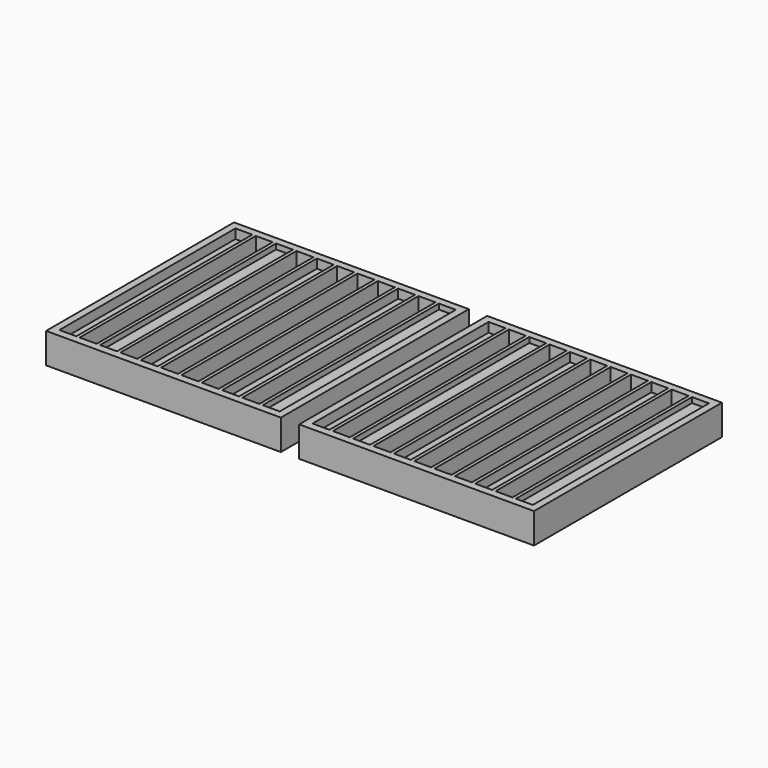
from build123d import *

# Parameters (mm, degrees)
F0_W     = 44.6
F0_H     = 55.1762282848
F0_H_2   = 34.8895229399
F0_H_3   = 66.0242550075
F0_H_4   = 3.5007570405
F0_H_5   = 56.2235750258
F0_H_6   = 10.0867319852
F1_DEPTH = 580
F0_H_7   = 24.8237717152
F0_H_8   = 45.1104770601
F0_H_9   = 13.9757449925
F0_H_10  = 76.4992429595
F0_H_11  = 23.7764249742
F0_H_12  = 69.9132680148
F2_DEPTH = 9
F3_START = 580
F3_DEPTH = 10
F4_W     = 618.6
F4_H     = 619
F4_W_2   = 598.6
F4_H_2   = 599
F5_DEPTH = 80


# Not quite as in the source:
# - a feature names something its author has since deleted; it is built from what else it names


with BuildPart() as f1:
    # F0 (on Front) → F1 (new body)
    with BuildSketch(Plane.XZ):
        Polygon((0, 80), (0, 0), (9, 0), (9, 55.1762282848), (9, 80), align=None)
        with Locations((31.3, 27.5881141424)):
            Rectangle(F0_W, F0_H)
        Polygon((53.6, 55.1762282848), (53.6, 0), (62.6, 0), (62.6, 34.8895229399), (62.6, 80), (53.6, 80), align=None)
        with Locations((84.9, 17.44476147)):
            Rectangle(F0_W, F0_H_2)
        Polygon((107.2, 34.8895229399), (107.2, 0), (116.2, 0), (116.2, 66.0242550075), (116.2, 80), (107.2, 80), align=None)
        with Locations((138.5, 33.0121275038)):
            Rectangle(F0_W, F0_H_3)
        Polygon((160.8, 66.0242550075), (160.8, 0), (169.8, 0), (169.8, 3.5007570405), (169.8, 80), (160.8, 80), align=None)
        with Locations((192.1, 1.7503785202)):
            Rectangle(F0_W, F0_H_4)
        Polygon((214.4, 3.5007570405), (214.4, 0), (223.4, 0), (223.4, 56.2235750258), (223.4, 80), (214.4, 80), align=None)
        with Locations((245.7, 28.1117875129)):
            Rectangle(F0_W, F0_H_5)
        Polygon((268, 56.2235750258), (268, 0), (277, 0), (277, 10.0867319852), (277, 80), (268, 80), align=None)
        with Locations((299.3, 5.0433659926)):
            Rectangle(F0_W, F0_H_6)
        Polygon((321.6, 10.0867319852), (321.6, 0), (330.6, 0), (330.6, 34.8895229399), (330.6, 80), (321.6, 80), align=None)
        with Locations((352.9, 17.44476147)):
            Rectangle(F0_W, F0_H_2)
        Polygon((375.2, 34.8895229399), (375.2, 0), (384.2, 0), (384.2, 10.0867319852), (384.2, 80), (375.2, 80), align=None)
        with Locations((406.5, 5.0433659926)):
            Rectangle(F0_W, F0_H_6)
        Polygon((428.8, 10.0867319852), (428.8, 0), (437.8, 0), (437.8, 56.2235750258), (437.8, 80), (428.8, 80), align=None)
        with Locations((460.1, 28.1117875129)):
            Rectangle(F0_W, F0_H_5)
        Polygon((482.4, 56.2235750258), (482.4, 0), (491.4, 0), (491.4, 3.5007570405), (491.4, 80), (482.4, 80), align=None)
        with Locations((513.7, 1.7503785202)):
            Rectangle(F0_W, F0_H_4)
        Polygon((536, 3.5007570405), (536, 0), (545, 0), (545, 66.0242550075), (545, 80), (536, 80), align=None)
        with Locations((567.3, 33.0121275038)):
            Rectangle(F0_W, F0_H_3)
        Polygon((589.6, 66.0242550075), (589.6, 0), (598.6, 0), (598.6, 80), (589.6, 80), align=None)
    extrude(amount=F1_DEPTH)

    # F0 (on Front) → F2 (join)
    with BuildSketch(Plane.XZ):
        Polygon((0, 80), (0, 0), (9, 0), (9, 55.1762282848), (9, 80), align=None)
        with Locations((31.3, 27.5881141424)):
            Rectangle(F0_W, F0_H)
        with Locations((31.3, 67.5881141424)):
            Rectangle(F0_W, F0_H_7)
        Polygon((53.6, 55.1762282848), (53.6, 0), (62.6, 0), (62.6, 34.8895229399), (62.6, 80), (53.6, 80), align=None)
        with Locations((84.9, 17.44476147)):
            Rectangle(F0_W, F0_H_2)
        with Locations((84.9, 57.44476147)):
            Rectangle(F0_W, F0_H_8)
        Polygon((107.2, 34.8895229399), (107.2, 0), (116.2, 0), (116.2, 66.0242550075), (116.2, 80), (107.2, 80), align=None)
        with Locations((138.5, 33.0121275038)):
            Rectangle(F0_W, F0_H_3)
        with Locations((138.5, 73.0121275038)):
            Rectangle(F0_W, F0_H_9)
        Polygon((160.8, 66.0242550075), (160.8, 0), (169.8, 0), (169.8, 3.5007570405), (169.8, 80), (160.8, 80), align=None)
        with Locations((192.1, 1.7503785202)):
            Rectangle(F0_W, F0_H_4)
        with Locations((192.1, 41.7503785202)):
            Rectangle(F0_W, F0_H_10)
        Polygon((214.4, 3.5007570405), (214.4, 0), (223.4, 0), (223.4, 56.2235750258), (223.4, 80), (214.4, 80), align=None)
        with Locations((245.7, 28.1117875129)):
            Rectangle(F0_W, F0_H_5)
        with Locations((245.7, 68.1117875129)):
            Rectangle(F0_W, F0_H_11)
        Polygon((268, 56.2235750258), (268, 0), (277, 0), (277, 10.0867319852), (277, 80), (268, 80), align=None)
        with Locations((299.3, 5.0433659926)):
            Rectangle(F0_W, F0_H_6)
        with Locations((299.3, 45.0433659926)):
            Rectangle(F0_W, F0_H_12)
        Polygon((321.6, 10.0867319852), (321.6, 0), (330.6, 0), (330.6, 34.8895229399), (330.6, 80), (321.6, 80), align=None)
        with Locations((352.9, 17.44476147)):
            Rectangle(F0_W, F0_H_2)
        with Locations((352.9, 57.44476147)):
            Rectangle(F0_W, F0_H_8)
        Polygon((375.2, 34.8895229399), (375.2, 0), (384.2, 0), (384.2, 10.0867319852), (384.2, 80), (375.2, 80), align=None)
        with Locations((406.5, 5.0433659926)):
            Rectangle(F0_W, F0_H_6)
        with Locations((406.5, 45.0433659926)):
            Rectangle(F0_W, F0_H_12)
        Polygon((428.8, 10.0867319852), (428.8, 0), (437.8, 0), (437.8, 56.2235750258), (437.8, 80), (428.8, 80), align=None)
        with Locations((460.1, 28.1117875129)):
            Rectangle(F0_W, F0_H_5)
        with Locations((460.1, 68.1117875129)):
            Rectangle(F0_W, F0_H_11)
        Polygon((482.4, 56.2235750258), (482.4, 0), (491.4, 0), (491.4, 3.5007570405), (491.4, 80), (482.4, 80), align=None)
        with Locations((513.7, 1.7503785202)):
            Rectangle(F0_W, F0_H_4)
        with Locations((513.7, 41.7503785202)):
            Rectangle(F0_W, F0_H_10)
        Polygon((536, 3.5007570405), (536, 0), (545, 0), (545, 66.0242550075), (545, 80), (536, 80), align=None)
        with Locations((567.3, 33.0121275038)):
            Rectangle(F0_W, F0_H_3)
        with Locations((567.3, 73.0121275038)):
            Rectangle(F0_W, F0_H_9)
        Polygon((589.6, 66.0242550075), (589.6, 0), (598.6, 0), (598.6, 80), (589.6, 80), align=None)
    extrude(amount=-F2_DEPTH)

    # F0 (on Front) → F3 (join)
    with BuildSketch(Plane.XZ.offset(F3_START)):
        Polygon((0, 80), (0, 0), (9, 0), (9, 55.1762282848), (9, 80), align=None)
        with Locations((31.3, 27.5881141424)):
            Rectangle(F0_W, F0_H)
        with Locations((31.3, 67.5881141424)):
            Rectangle(F0_W, F0_H_7)
        Polygon((53.6, 55.1762282848), (53.6, 0), (62.6, 0), (62.6, 34.8895229399), (62.6, 80), (53.6, 80), align=None)
        with Locations((84.9, 17.44476147)):
            Rectangle(F0_W, F0_H_2)
        with Locations((84.9, 57.44476147)):
            Rectangle(F0_W, F0_H_8)
        Polygon((107.2, 34.8895229399), (107.2, 0), (116.2, 0), (116.2, 66.0242550075), (116.2, 80), (107.2, 80), align=None)
        with Locations((138.5, 33.0121275038)):
            Rectangle(F0_W, F0_H_3)
        with Locations((138.5, 73.0121275038)):
            Rectangle(F0_W, F0_H_9)
        Polygon((160.8, 66.0242550075), (160.8, 0), (169.8, 0), (169.8, 3.5007570405), (169.8, 80), (160.8, 80), align=None)
        with Locations((192.1, 1.7503785202)):
            Rectangle(F0_W, F0_H_4)
        with Locations((192.1, 41.7503785202)):
            Rectangle(F0_W, F0_H_10)
        Polygon((214.4, 3.5007570405), (214.4, 0), (223.4, 0), (223.4, 56.2235750258), (223.4, 80), (214.4, 80), align=None)
        with Locations((245.7, 28.1117875129)):
            Rectangle(F0_W, F0_H_5)
        with Locations((245.7, 68.1117875129)):
            Rectangle(F0_W, F0_H_11)
        Polygon((268, 56.2235750258), (268, 0), (277, 0), (277, 10.0867319852), (277, 80), (268, 80), align=None)
        with Locations((299.3, 5.0433659926)):
            Rectangle(F0_W, F0_H_6)
        with Locations((299.3, 45.0433659926)):
            Rectangle(F0_W, F0_H_12)
        Polygon((321.6, 10.0867319852), (321.6, 0), (330.6, 0), (330.6, 34.8895229399), (330.6, 80), (321.6, 80), align=None)
        with Locations((352.9, 17.44476147)):
            Rectangle(F0_W, F0_H_2)
        with Locations((352.9, 57.44476147)):
            Rectangle(F0_W, F0_H_8)
        Polygon((375.2, 34.8895229399), (375.2, 0), (384.2, 0), (384.2, 10.0867319852), (384.2, 80), (375.2, 80), align=None)
        with Locations((406.5, 5.0433659926)):
            Rectangle(F0_W, F0_H_6)
        with Locations((406.5, 45.0433659926)):
            Rectangle(F0_W, F0_H_12)
        Polygon((428.8, 10.0867319852), (428.8, 0), (437.8, 0), (437.8, 56.2235750258), (437.8, 80), (428.8, 80), align=None)
        with Locations((460.1, 28.1117875129)):
            Rectangle(F0_W, F0_H_5)
        with Locations((460.1, 68.1117875129)):
            Rectangle(F0_W, F0_H_11)
        Polygon((482.4, 56.2235750258), (482.4, 0), (491.4, 0), (491.4, 3.5007570405), (491.4, 80), (482.4, 80), align=None)
        with Locations((513.7, 1.7503785202)):
            Rectangle(F0_W, F0_H_4)
        with Locations((513.7, 41.7503785202)):
            Rectangle(F0_W, F0_H_10)
        Polygon((536, 3.5007570405), (536, 0), (545, 0), (545, 66.0242550075), (545, 80), (536, 80), align=None)
        with Locations((567.3, 33.0121275038)):
            Rectangle(F0_W, F0_H_3)
        with Locations((567.3, 73.0121275038)):
            Rectangle(F0_W, F0_H_9)
        Polygon((589.6, 66.0242550075), (589.6, 0), (598.6, 0), (598.6, 80), (589.6, 80), align=None)
    extrude(amount=F3_DEPTH)

    # F4 (on face) → F5 (join, through all)
    with BuildSketch(Plane.XY.offset(80)):
        with Locations((299.3, -290.5)):
            Rectangle(F4_W, F4_H)
        with Locations((299.3, -290.5)):
            Rectangle(F4_W_2, F4_H_2, mode=Mode.SUBTRACT)
    extrude(amount=-F5_DEPTH)


with BuildPart() as f6_1:
    # F6: copy of F1
    add(f1.part.moved(Location((667, 0, 0))))


solid = Compound([f1.part, f6_1.part])
